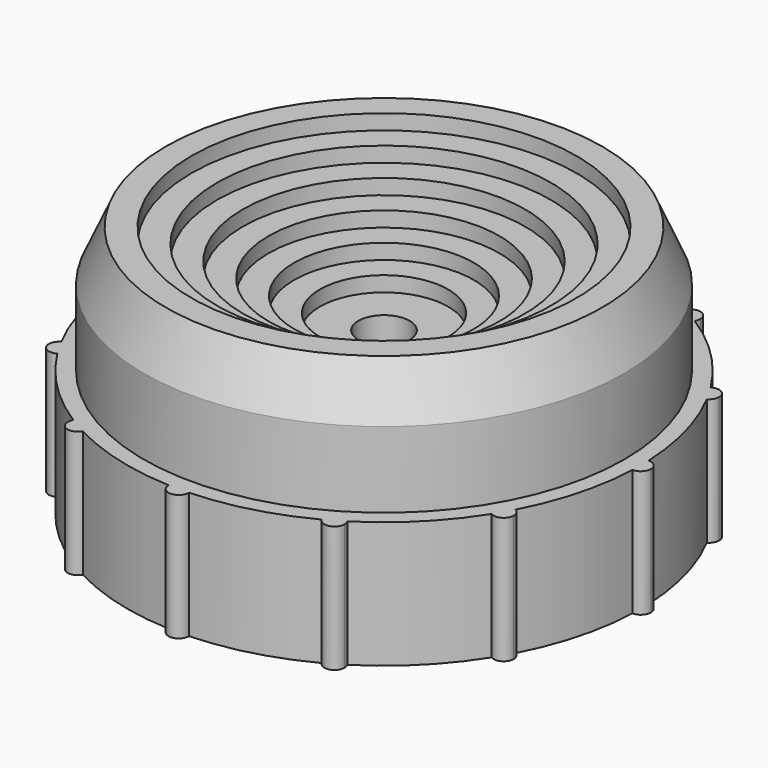
from build123d import *

# Parameters (mm, degrees)
F3_DEPTH = 12.5
F2_R     = 6.477
F4_DEPTH = 7.62
F5_R     = 2.54
F6_DEPTH = 25.4


with BuildPart() as f1:
    # F0 (on Front) → F1 (revolve)
    with BuildSketch(Plane.XZ):
        Polygon((-25.4, 0), (0, 0), (0, 16), (-6.35, 16), (-6.35, 17.5), (-8.89, 17.5), (-8.89, 19), (-11.43, 19), (-11.43, 20.5), (-13.97, 20.5), (-13.97, 22), (-16.51, 22), (-16.51, 23.5), (-19.05, 23.5), (-19.05, 25), (-21.59, 25), (-23.8, 20), (-23.8, 12.5), (-25.4, 12.5), align=None)
    revolve(axis=Axis((0, 0, 8), (0, 0, -1)))

    # F2 (on face) → F3 (join)
    with BuildSketch(Plane(origin=(0, 0, 0), x_dir=(1, 0, 0), z_dir=(0, 0, -1))):
        with BuildLine():
            ThreePointArc((-25.3803149606, -0.9998062308), (-25.4, 0), (-25.3803149606, 0.9998062308))
            ThreePointArc((-25.3803149606, 0.9998062308), (-26.4, 0), (-25.3803149606, -0.9998062308))
        make_face()
        with BuildLine():
            ThreePointArc((-21.4800943965, 13.5560150751), (-21.9970452561, 12.7), (-22.4799006274, 11.8242998855))
            ThreePointArc((-22.4799006274, 11.8242998855), (-21.4885451928, 11.8389380477), (-20.9970452561, 12.7))
            ThreePointArc((-20.9970452561, 12.7), (-21.1261403074, 13.1914514932), (-21.4800943965, 13.5560150751))
        make_face()
        with BuildLine():
            ThreePointArc((-21.4800943965, 13.5560150751), (-22.8630706599, 13.2), (-22.4799006274, 11.8242998855))
            ThreePointArc((-22.4799006274, 11.8242998855), (-21.9970452561, 12.7), (-21.4800943965, 13.5560150751))
        make_face()
        with BuildLine():
            ThreePointArc((-21.4800943965, -13.5560150751), (-21.9970452561, -12.7), (-22.4799006274, -11.8242998855))
            ThreePointArc((-22.4799006274, -11.8242998855), (-22.8630706599, -13.2), (-21.4800943965, -13.5560150751))
        make_face()
        with BuildLine():
            ThreePointArc((-11.8242998855, 22.4799006274), (-12.7, 21.9970452561), (-13.5560150751, 21.4800943965))
            ThreePointArc((-13.5560150751, 21.4800943965), (-12.4316858884, 21.0337137776), (-11.7, 21.9970452561))
            ThreePointArc((-11.7, 21.9970452561), (-11.7315734115, 22.2463441586), (-11.8242998855, 22.4799006274))
        make_face()
        with BuildLine():
            ThreePointArc((-11.8242998855, 22.4799006274), (-13.2, 22.8630706599), (-13.5560150751, 21.4800943965))
            ThreePointArc((-13.5560150751, 21.4800943965), (-12.7, 21.9970452561), (-11.8242998855, 22.4799006274))
        make_face()
        with BuildLine():
            ThreePointArc((-11.8242998855, -22.4799006274), (-12.7, -21.9970452561), (-13.5560150751, -21.4800943965))
            ThreePointArc((-13.5560150751, -21.4800943965), (-13.2, -22.8630706599), (-11.8242998855, -22.4799006274))
        make_face()
        with BuildLine():
            ThreePointArc((0.9998062308, 25.3803149606), (0, 25.4), (-0.9998062308, 25.3803149606))
            ThreePointArc((-0.9998062308, 25.3803149606), (0, 24.4), (0.9998062308, 25.3803149606))
        make_face()
        with BuildLine():
            ThreePointArc((1, 25.4), (-0.0098429965, 26.3999515565), (-0.9998062308, 25.3803149606))
            ThreePointArc((-0.9998062308, 25.3803149606), (0, 25.4), (0.9998062308, 25.3803149606))
            ThreePointArc((0.9998062308, 25.3803149606), (0.9999515565, 25.3901570035), (1, 25.4))
        make_face()
        with BuildLine():
            ThreePointArc((0.9998062308, -25.3803149606), (0, -25.4), (-0.9998062308, -25.3803149606))
            ThreePointArc((-0.9998062308, -25.3803149606), (-0.0098429965, -26.3999515565), (1, -25.4))
            ThreePointArc((1, -25.4), (0.9999515565, -25.3901570035), (0.9998062308, -25.3803149606))
        make_face()
        with BuildLine():
            ThreePointArc((13.5560150751, 21.4800943965), (12.7, 21.9970452561), (11.8242998855, 22.4799006274))
            ThreePointArc((11.8242998855, 22.4799006274), (12.2, 21.1310198523), (13.5560150751, 21.4800943965))
        make_face()
        with BuildLine():
            ThreePointArc((13.7, 21.9970452561), (12.9492989025, 22.9654718446), (11.8242998855, 22.4799006274))
            ThreePointArc((11.8242998855, 22.4799006274), (12.7, 21.9970452561), (13.5560150751, 21.4800943965))
            ThreePointArc((13.5560150751, 21.4800943965), (13.6633314785, 21.7287311446), (13.7, 21.9970452561))
        make_face()
        with BuildLine():
            ThreePointArc((13.5560150751, -21.4800943965), (12.7, -21.9970452561), (11.8242998855, -22.4799006274))
            ThreePointArc((11.8242998855, -22.4799006274), (12.9492989025, -22.9654718446), (13.7, -21.9970452561))
            ThreePointArc((13.7, -21.9970452561), (13.6633314785, -21.7287311446), (13.5560150751, -21.4800943965))
        make_face()
        with BuildLine():
            ThreePointArc((22.4799006274, 11.8242998855), (21.9970452561, 12.7), (21.4800943965, 13.5560150751))
            ThreePointArc((21.4800943965, 13.5560150751), (21.1310198523, 12.2), (22.4799006274, 11.8242998855))
        make_face()
        with BuildLine():
            ThreePointArc((22.9970452561, 12.7), (22.4884967494, 13.5709049488), (21.4800943965, 13.5560150751))
            ThreePointArc((21.4800943965, 13.5560150751), (21.9970452561, 12.7), (22.4799006274, 11.8242998855))
            ThreePointArc((22.4799006274, 11.8242998855), (22.8581072084, 12.1914999367), (22.9970452561, 12.7))
        make_face()
        with BuildLine():
            ThreePointArc((22.4799006274, -11.8242998855), (21.9970452561, -12.7), (21.4800943965, -13.5560150751))
            ThreePointArc((21.4800943965, -13.5560150751), (22.4884967494, -13.5709049488), (22.9970452561, -12.7))
            ThreePointArc((22.9970452561, -12.7), (22.8581072084, -12.1914999367), (22.4799006274, -11.8242998855))
        make_face()
        with BuildLine():
            ThreePointArc((26.4, 0), (26.1001124769, 0.7140325761), (25.3803149606, 0.9998062308))
            ThreePointArc((25.3803149606, 0.9998062308), (25.3950782633, 0.5), (25.4, 0))
            ThreePointArc((25.4, 0), (25.3950782633, -0.5), (25.3803149606, -0.9998062308))
            ThreePointArc((25.3803149606, -0.9998062308), (26.1001124769, -0.7140325761), (26.4, 0))
        make_face()
    extrude(amount=-F3_DEPTH)

    # F2 (on face) → F4 (cut)
    with BuildSketch(Plane(origin=(0, 0, 0), x_dir=(1, 0, 0), z_dir=(0, 0, -1))):
        Circle(F2_R)
    extrude(amount=-F4_DEPTH, mode=Mode.SUBTRACT)

    # F5 (on face) → F6 (cut)
    with BuildSketch(Plane.XY.offset(16)):
        Circle(F5_R)
    extrude(amount=-F6_DEPTH, mode=Mode.SUBTRACT)


solid = f1.part
